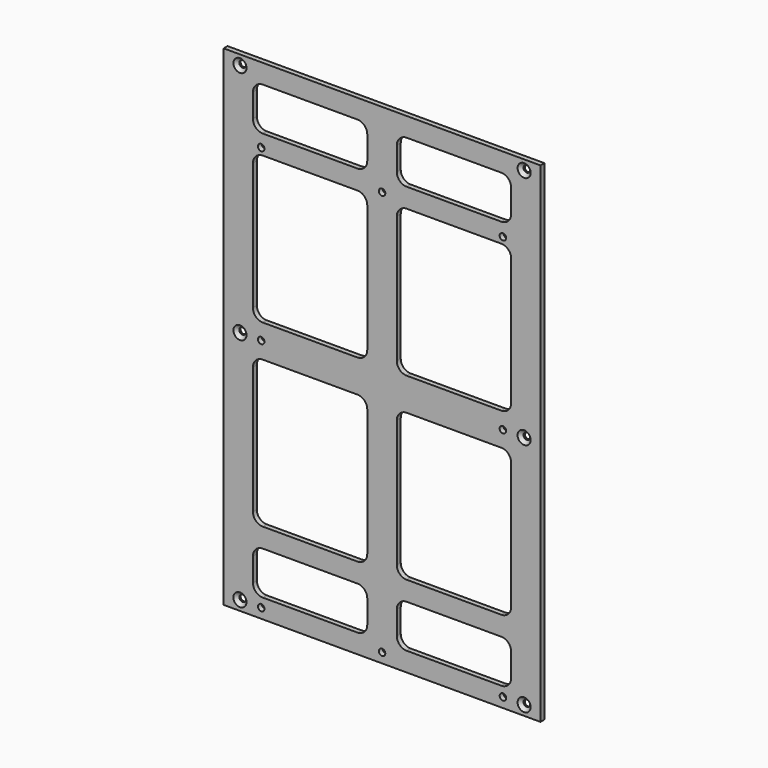
from build123d import *

# Parameters (mm, degrees)
F0_W           = 97
F0_H           = 150
F1_DEPTH       = 1.5
F3_D           = 2
F3_CSINK_D     = 4
F3_CSINK_ANGLE = 90
F5_D           = 2


# Not quite as in the source:
# - a feature names something its author has since deleted; it is built from what else it names


with BuildPart() as f1:
    # F0 (on Front) → F1 (new body)
    with BuildSketch(Plane.XZ):
        Rectangle(F0_W, F0_H)
        with BuildLine():
            Line((-4.5249225795, -58.9309873283), (-4.5249225795, -66.1341202259))
            ThreePointArc((-4.5249225795, -66.1341202259), (-5.403602236, -68.2554405695), (-7.5249225795, -69.1341202259))
            Line((-7.5249225795, -69.1341202259), (-36.5249225795, -69.1341202259))
            ThreePointArc((-36.5249225795, -69.1341202259), (-38.6462429231, -68.2554405695), (-39.5249225795, -66.1341202259))
            Line((-39.5249225795, -66.1341202259), (-39.5249225795, -58.9309873283))
            ThreePointArc((-39.5249225795, -58.9309873283), (-38.6462429231, -56.8096669847), (-36.5249225795, -55.9309873283))
            Line((-36.5249225795, -55.9309873283), (-7.5249225795, -55.9309873283))
            ThreePointArc((-7.5249225795, -55.9309873283), (-5.403602236, -56.8096669847), (-4.5249225795, -58.9309873283))
        make_face(mode=Mode.SUBTRACT)
        with BuildLine():
            Line((-36.5249225795, -5), (-7.5249225795, -5))
            ThreePointArc((-7.5249225795, -5), (-5.403602236, -5.8786796564), (-4.5249225795, -8))
            Line((-4.5249225795, -8), (-4.5249225795, -47))
            ThreePointArc((-4.5249225795, -47), (-5.403602236, -49.1213203436), (-7.5249225795, -50))
            Line((-7.5249225795, -50), (-36.5249225795, -50))
            ThreePointArc((-36.5249225795, -50), (-38.6462429231, -49.1213203436), (-39.5249225795, -47))
            Line((-39.5249225795, -47), (-39.5249225795, -8))
            ThreePointArc((-39.5249225795, -8), (-38.6462429231, -5.8786796564), (-36.5249225795, -5))
        make_face(mode=Mode.SUBTRACT)
        with BuildLine():
            ThreePointArc((4.5249225795, -58.9309873283), (5.403602236, -56.8096669847), (7.5249225795, -55.9309873283))
            Line((7.5249225795, -55.9309873283), (36.5249225795, -55.9309873283))
            ThreePointArc((36.5249225795, -55.9309873283), (38.6462429231, -56.8096669847), (39.5249225795, -58.9309873283))
            Line((39.5249225795, -58.9309873283), (39.5249225795, -66.1341202259))
            ThreePointArc((39.5249225795, -66.1341202259), (38.6462429231, -68.2554405695), (36.5249225795, -69.1341202259))
            Line((36.5249225795, -69.1341202259), (7.5249225795, -69.1341202259))
            ThreePointArc((7.5249225795, -69.1341202259), (5.403602236, -68.2554405695), (4.5249225795, -66.1341202259))
            Line((4.5249225795, -66.1341202259), (4.5249225795, -58.9309873283))
        make_face(mode=Mode.SUBTRACT)
        with BuildLine():
            ThreePointArc((39.5249225795, -47), (38.6462429231, -49.1213203436), (36.5249225795, -50))
            Line((36.5249225795, -50), (7.5249225795, -50))
            ThreePointArc((7.5249225795, -50), (5.403602236, -49.1213203436), (4.5249225795, -47))
            Line((4.5249225795, -47), (4.5249225795, -8))
            ThreePointArc((4.5249225795, -8), (5.403602236, -5.8786796564), (7.5249225795, -5))
            Line((7.5249225795, -5), (36.5249225795, -5))
            ThreePointArc((36.5249225795, -5), (38.6462429231, -5.8786796564), (39.5249225795, -8))
            Line((39.5249225795, -8), (39.5249225795, -47))
        make_face(mode=Mode.SUBTRACT)
        with BuildLine():
            ThreePointArc((-4.5249225795, 8), (-5.403602236, 5.8786796564), (-7.5249225795, 5))
            Line((-7.5249225795, 5), (-36.5249225795, 5))
            ThreePointArc((-36.5249225795, 5), (-38.6462429231, 5.8786796564), (-39.5249225795, 8))
            Line((-39.5249225795, 8), (-39.5249225795, 47))
            ThreePointArc((-39.5249225795, 47), (-38.6462429231, 49.1213203436), (-36.5249225795, 50))
            Line((-36.5249225795, 50), (-7.5249225795, 50))
            ThreePointArc((-7.5249225795, 50), (-5.403602236, 49.1213203436), (-4.5249225795, 47))
            Line((-4.5249225795, 47), (-4.5249225795, 8))
        make_face(mode=Mode.SUBTRACT)
        with BuildLine():
            ThreePointArc((-4.5249225795, 58.9309873283), (-5.403602236, 56.8096669847), (-7.5249225795, 55.9309873283))
            Line((-7.5249225795, 55.9309873283), (-36.5249225795, 55.9309873283))
            ThreePointArc((-36.5249225795, 55.9309873283), (-38.6462429231, 56.8096669847), (-39.5249225795, 58.9309873283))
            Line((-39.5249225795, 58.9309873283), (-39.5249225795, 66.1341202259))
            ThreePointArc((-39.5249225795, 66.1341202259), (-38.6462429231, 68.2554405695), (-36.5249225795, 69.1341202259))
            Line((-36.5249225795, 69.1341202259), (-7.5249225795, 69.1341202259))
            ThreePointArc((-7.5249225795, 69.1341202259), (-5.403602236, 68.2554405695), (-4.5249225795, 66.1341202259))
            Line((-4.5249225795, 66.1341202259), (-4.5249225795, 58.9309873283))
        make_face(mode=Mode.SUBTRACT)
        with BuildLine():
            ThreePointArc((7.5249225795, 5), (5.403602236, 5.8786796564), (4.5249225795, 8))
            Line((4.5249225795, 8), (4.5249225795, 47))
            ThreePointArc((4.5249225795, 47), (5.403602236, 49.1213203436), (7.5249225795, 50))
            Line((7.5249225795, 50), (36.5249225795, 50))
            ThreePointArc((36.5249225795, 50), (38.6462429231, 49.1213203436), (39.5249225795, 47))
            Line((39.5249225795, 47), (39.5249225795, 8))
            ThreePointArc((39.5249225795, 8), (38.6462429231, 5.8786796564), (36.5249225795, 5))
            Line((36.5249225795, 5), (7.5249225795, 5))
        make_face(mode=Mode.SUBTRACT)
        with BuildLine():
            Line((7.5249225795, 69.1341202259), (36.5249225795, 69.1341202259))
            ThreePointArc((36.5249225795, 69.1341202259), (38.6462429231, 68.2554405695), (39.5249225795, 66.1341202259))
            Line((39.5249225795, 66.1341202259), (39.5249225795, 58.9309873283))
            ThreePointArc((39.5249225795, 58.9309873283), (38.6462429231, 56.8096669847), (36.5249225795, 55.9309873283))
            Line((36.5249225795, 55.9309873283), (7.5249225795, 55.9309873283))
            ThreePointArc((7.5249225795, 55.9309873283), (5.403602236, 56.8096669847), (4.5249225795, 58.9309873283))
            Line((4.5249225795, 58.9309873283), (4.5249225795, 66.1341202259))
            ThreePointArc((4.5249225795, 66.1341202259), (5.403602236, 68.2554405695), (7.5249225795, 69.1341202259))
        make_face(mode=Mode.SUBTRACT)
    extrude(amount=F1_DEPTH)

    # F3 (through all)
    with Locations(Plane.XZ.offset(1.5)):
        with Locations((-43.5, -72), (43.5, -72), (43.5, 72), (-43.5, 72), (-43.5, 0), (43.5, 0)):
            CounterSinkHole(F3_D / 2, F3_CSINK_D / 2, counter_sink_angle=F3_CSINK_ANGLE)

    # F5 (through all)
    with Locations(Plane.XZ.offset(1.5)):
        with Locations((-37, -72), (0, -72), (37, -72), (0, 52), (-37, 52), (37, 52), (-37, 0), (37, 0)):
            Hole(F5_D / 2)


solid = f1.part
